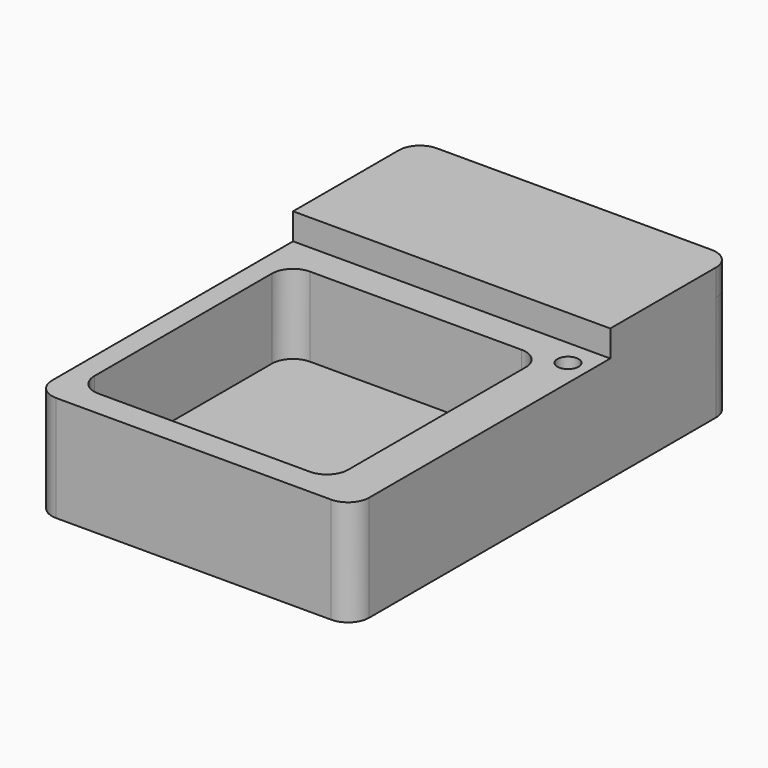
from build123d import *

# Parameters (mm, degrees)
F0_W     = 76.2
F0_H     = 114.3
F0_R     = 2.54
F1_DEPTH = 12.7
F2_R     = 5.08
F4_DEPTH = 6.35
F5_W     = 60.96
F5_H     = 63.5
F6_DEPTH = 19.05
F7_R     = 5.08


with BuildPart() as f1:
    # F0 (on Top) → F1 (new body, symmetric)
    with BuildSketch(Plane.XY):
        Rectangle(F0_W, F0_H)
        with Locations((33.02, 13.97)):
            Circle(F0_R, mode=Mode.SUBTRACT)
    extrude(amount=F1_DEPTH, both=True)

    # F2
    f2_edges = [f1.edges().sort_by_distance(p)[0] for p in [
        (-38.1, -57.15, 0),
        (38.1, -57.15, 0),
        (-38.1, 57.15, 0),
        (38.1, 57.15, 0),
    ]]
    fillet(f2_edges, radius=F2_R)

    # F3 (on face) → F4 (join)
    with BuildSketch(Plane.XY.offset(12.7)):
        with BuildLine():
            Line((-33.02, 57.15), (-38.1, 57.15))
            Line((-38.1, 57.15), (-38.1, 52.07))
            ThreePointArc((-38.1, 52.07), (-36.6121024484, 55.6621024484), (-33.02, 57.15))
        make_face()
        with BuildLine():
            Line((33.02, 57.15), (-33.02, 57.15))
            ThreePointArc((-33.02, 57.15), (-36.6121024484, 55.6621024484), (-38.1, 52.07))
            Line((-38.1, 52.07), (-38.1, 20.32))
            Line((-38.1, 20.32), (38.1, 20.32))
            Line((38.1, 20.32), (38.1, 52.07))
            ThreePointArc((38.1, 52.07), (36.6121024484, 55.6621024484), (33.02, 57.15))
        make_face()
        with BuildLine():
            Line((38.1, 57.15), (33.02, 57.15))
            ThreePointArc((33.02, 57.15), (36.6121024484, 55.6621024484), (38.1, 52.07))
            Line((38.1, 52.07), (38.1, 57.15))
        make_face()
    extrude(amount=F4_DEPTH)

    # F5 (on face) → F6 (cut)
    with BuildSketch(Plane.XY.offset(12.7)):
        with Locations((-2.54, -19.05)):
            Rectangle(F5_W, F5_H)
    extrude(amount=-F6_DEPTH, mode=Mode.SUBTRACT)

    # F7
    f7_edges = [f1.edges().sort_by_distance(p)[0] for p in [
        (-33.02, 12.7, 3.175),
        (-33.02, -50.8, 3.175),
        (27.94, 12.7, 3.175),
        (27.94, -50.8, 3.175),
        (-38.1, 57.15, 15.875),
        (38.1, 57.15, 15.875),
    ]]
    fillet(f7_edges, radius=F7_R)


solid = f1.part
